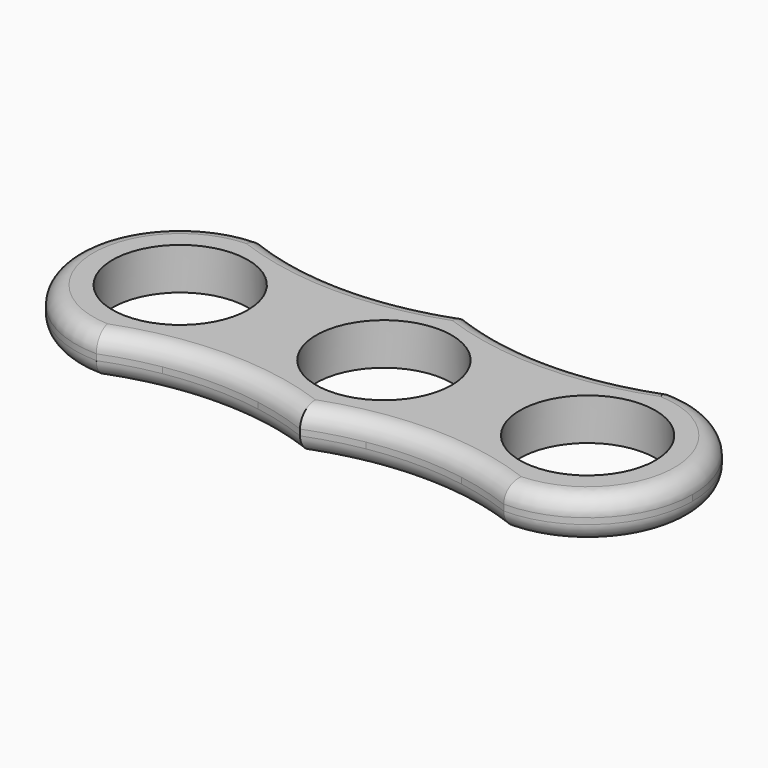
from build123d import *

# Parameters (mm, degrees)
F0_R         = 11.3
F1_DEPTH     = 7
F2_T2_ANGLE  = 60.8488693261
F2_T4_ANGLE  = 229.1896473945
F2_T6_ANGLE  = 60.8488693261
F2_T8_ANGLE  = 60.8488693262
F2_T10_ANGLE = 229.1896473945
F2_T12_ANGLE = 60.8488693262
F3_T2_ANGLE  = 60.8488693261
F3_T4_ANGLE  = 229.1896473945
F3_T6_ANGLE  = 60.8488693261
F3_T8_ANGLE  = 60.8488693262
F3_T10_ANGLE = 60.8488693262
F3_T12_ANGLE = 229.1896473945


# Not quite as in the source:
# - a fillet or chamfer that OpenCascade refuses, or shapes differently, is made with other operations: its cross-section is extruded or revolved along the edge and cut away or added


with BuildPart() as f1:
    # F0 (on Top) → F1 (new body)
    with BuildSketch(Plane.XY):
        with BuildLine():
            ThreePointArc((17, -4.1533119315), (17.3745503539, -2.0916500663), (17.5, 0))
            ThreePointArc((17.5, 0), (17.3745503539, 2.0916500663), (17, 4.1533119315))
            ThreePointArc((17, 4.1533119315), (16.5, 0), (17, -4.1533119315))
        make_face()
        with BuildLine():
            ThreePointArc((17, 4.1533119315), (17.3745503539, 2.0916500663), (17.5, 0))
            ThreePointArc((17.5, 0), (17.3745503539, -2.0916500663), (17, -4.1533119315))
            ThreePointArc((17, -4.1533119315), (19.903404144, -10.3699558954), (24.9737217118, -14.9925414878))
            ThreePointArc((24.9737217118, -14.9925414878), (29.5496426675, -16.0202705528), (34, -17.5))
            ThreePointArc((34, -17.5), (46.3743686708, -12.3743686708), (51.5, 0))
            ThreePointArc((51.5, 0), (46.3743686708, 12.3743686708), (34, 17.5))
            ThreePointArc((34, 17.5), (29.5496426675, 16.0202705528), (24.9737217118, 14.9925414878))
            ThreePointArc((24.9737217118, 14.9925414878), (19.903404144, 10.3699558954), (17, 4.1533119315))
        make_face()
        with Locations((34, 0)):
            Circle(F0_R, mode=Mode.SUBTRACT)
        with BuildLine():
            ThreePointArc((17, -4.1533119315), (16.5, 0), (17, 4.1533119315))
            ThreePointArc((17, 4.1533119315), (14.096595856, 10.3699558954), (9.0262782882, 14.9925414878))
            ThreePointArc((9.0262782882, 14.9925414878), (4.4503573325, 16.0202705528), (0, 17.5))
            ThreePointArc((0, 17.5), (-4.4503573325, 16.0202705528), (-9.0262782882, 14.9925414878))
            ThreePointArc((-9.0262782882, 14.9925414878), (-14.096595856, 10.3699558954), (-17, 4.1533119315))
            ThreePointArc((-17, 4.1533119315), (-16.6254496461, 2.0916500663), (-16.5, 0))
            ThreePointArc((-16.5, 0), (-16.6254496461, -2.0916500663), (-17, -4.1533119315))
            ThreePointArc((-17, -4.1533119315), (-14.096595856, -10.3699558954), (-9.0262782882, -14.9925414878))
            ThreePointArc((-9.0262782882, -14.9925414878), (-4.4503573325, -16.0202705528), (0, -17.5))
            ThreePointArc((0, -17.5), (4.4503573325, -16.0202705528), (9.0262782882, -14.9925414878))
            ThreePointArc((9.0262782882, -14.9925414878), (14.096595856, -10.3699558954), (17, -4.1533119315))
        make_face()
        Circle(F0_R, mode=Mode.SUBTRACT)
        with BuildLine():
            ThreePointArc((9.0262782882, 14.9925414878), (14.096595856, 10.3699558954), (17, 4.1533119315))
            ThreePointArc((17, 4.1533119315), (19.903404144, 10.3699558954), (24.9737217118, 14.9925414878))
            ThreePointArc((24.9737217118, 14.9925414878), (17, 14.3095450998), (9.0262782882, 14.9925414878))
        make_face()
        with BuildLine():
            ThreePointArc((24.9737217118, -14.9925414878), (19.903404144, -10.3699558954), (17, -4.1533119315))
            ThreePointArc((17, -4.1533119315), (14.096595856, -10.3699558954), (9.0262782882, -14.9925414878))
            ThreePointArc((9.0262782882, -14.9925414878), (17, -14.3095450998), (24.9737217118, -14.9925414878))
        make_face()
        with BuildLine():
            ThreePointArc((-17, 4.1533119315), (-14.096595856, 10.3699558954), (-9.0262782882, 14.9925414878))
            ThreePointArc((-9.0262782882, 14.9925414878), (-17, 14.3095450998), (-24.9737217118, 14.9925414878))
            ThreePointArc((-24.9737217118, 14.9925414878), (-19.903404144, 10.3699558954), (-17, 4.1533119315))
        make_face()
        with BuildLine():
            ThreePointArc((-24.9737217118, -14.9925414878), (-17, -14.3095450998), (-9.0262782882, -14.9925414878))
            ThreePointArc((-9.0262782882, -14.9925414878), (-14.096595856, -10.3699558954), (-17, -4.1533119315))
            ThreePointArc((-17, -4.1533119315), (-19.903404144, -10.3699558954), (-24.9737217118, -14.9925414878))
        make_face()
        with BuildLine():
            ThreePointArc((-16.5, 0), (-16.6254496461, 2.0916500663), (-17, 4.1533119315))
            ThreePointArc((-17, 4.1533119315), (-17.5, 0), (-17, -4.1533119315))
            ThreePointArc((-17, -4.1533119315), (-16.6254496461, -2.0916500663), (-16.5, 0))
        make_face()
        with BuildLine():
            ThreePointArc((-17, -4.1533119315), (-17.5, 0), (-17, 4.1533119315))
            ThreePointArc((-17, 4.1533119315), (-19.903404144, 10.3699558954), (-24.9737217118, 14.9925414878))
            ThreePointArc((-24.9737217118, 14.9925414878), (-29.5496426675, 16.0202705528), (-34, 17.5))
            ThreePointArc((-34, 17.5), (-51.5, 0), (-34, -17.5))
            ThreePointArc((-34, -17.5), (-29.5496426675, -16.0202705528), (-24.9737217118, -14.9925414878))
            ThreePointArc((-24.9737217118, -14.9925414878), (-19.903404144, -10.3699558954), (-17, -4.1533119315))
        make_face()
        with Locations((-34, 0)):
            Circle(F0_R, mode=Mode.SUBTRACT)
    extrude(amount=F1_DEPTH)

    # F2: fillet of radius 3 on 6 edges, made by hand

    # F2_s1 → F2_t2 (revolve, cut)
    with BuildSketch(Plane(origin=(-39.3629213467, -23.1166596288, 0), x_dir=(0, 0, 1), z_dir=(-0.8622977849, -0.5064015503, 0))):
        with BuildLine():
            ThreePointArc((4, 2.7261224717), (6.1213203436, 3.6048021282), (7, 5.7261224717))
            Line((7, 5.7261224717), (7, 2.7261224717))
            Line((7, 2.7261224717), (4, 2.7261224717))
        make_face()
    revolve(axis=Axis((-17, -61.1961195589, 7), (0, 0, -1)), revolution_arc=F2_T2_ANGLE, mode=Mode.SUBTRACT)

    # F2_s3 → F2_t4 (revolve, cut)
    with BuildSketch(Plane(origin=(-28.110475333, 12.8669086371, 0), x_dir=(0, 0, 1), z_dir=(0.9092737136, -0.416198647, 0))):
        with BuildLine():
            ThreePointArc((4, -3.3492460032), (6.1213203436, -2.4705663467), (7, -0.3492460032))
            Line((7, -0.3492460032), (7, -3.3492460032))
            Line((7, -3.3492460032), (4, -3.3492460032))
        make_face()
    revolve(axis=Axis((-34, 0, 7), (0, 0, 1)), revolution_arc=F2_T4_ANGLE, mode=Mode.SUBTRACT)

    # F2_s5 → F2_t6 (revolve, cut)
    with BuildSketch(Plane(origin=(14.0819673704, 8.2699158362, 0), x_dir=(0, 0, 1), z_dir=(0.8622977849, 0.5064015503, 0))):
        with BuildLine():
            ThreePointArc((4, -14.4915302372), (6.1213203436, -13.6128505808), (7, -11.4915302372))
            Line((7, -11.4915302372), (7, -14.4915302372))
            Line((7, -14.4915302372), (4, -14.4915302372))
        make_face()
    revolve(axis=Axis((-17, 61.1961195589, 7), (0, 0, -1)), revolution_arc=F2_T6_ANGLE, mode=Mode.SUBTRACT)

    # F2_s7 → F2_t8 (revolve, cut)
    with BuildSketch(Plane(origin=(39.3629213467, 23.1166596288, 0), x_dir=(0, 0, 1), z_dir=(0.8622977849, 0.5064015503, 0))):
        with BuildLine():
            ThreePointArc((4, 2.7261224717), (6.1213203436, 3.6048021282), (7, 5.7261224717))
            Line((7, 5.7261224717), (7, 2.7261224717))
            Line((7, 2.7261224717), (4, 2.7261224717))
        make_face()
    revolve(axis=Axis((17, 61.1961195588, 7), (0, 0, -1)), revolution_arc=F2_T8_ANGLE, mode=Mode.SUBTRACT)

    # F2_s9 → F2_t10 (revolve, cut)
    with BuildSketch(Plane(origin=(28.110475333, -12.8669086371, 0), x_dir=(0, 0, 1), z_dir=(-0.9092737136, 0.416198647, 0))):
        with BuildLine():
            ThreePointArc((4, -3.3492460032), (6.1213203436, -2.4705663467), (7, -0.3492460032))
            Line((7, -0.3492460032), (7, -3.3492460032))
            Line((7, -3.3492460032), (4, -3.3492460032))
        make_face()
    revolve(axis=Axis((34, 0, 7), (0, 0, 1)), revolution_arc=F2_T10_ANGLE, mode=Mode.SUBTRACT)

    # F2_s11 → F2_t12 (revolve, cut)
    with BuildSketch(Plane(origin=(-14.0819673704, -8.2699158362, 0), x_dir=(0, 0, 1), z_dir=(-0.8622977849, -0.5064015503, 0))):
        with BuildLine():
            ThreePointArc((4, -14.4915302372), (6.1213203436, -13.6128505808), (7, -11.4915302372))
            Line((7, -11.4915302372), (7, -14.4915302372))
            Line((7, -14.4915302372), (4, -14.4915302372))
        make_face()
    revolve(axis=Axis((17, -61.1961195588, 7), (0, 0, -1)), revolution_arc=F2_T12_ANGLE, mode=Mode.SUBTRACT)

    # F3: fillet of radius 3 on 6 edges, made by hand

    # F3_s1 → F3_t2 (revolve, cut)
    with BuildSketch(Plane(origin=(-39.3629213467, -23.1166596288, 0), x_dir=(0, 0, 1), z_dir=(-0.8622977849, -0.5064015503, 0))):
        with BuildLine():
            ThreePointArc((0, 5.7261224717), (0.8786796564, 3.6048021282), (3, 2.7261224717))
            Line((3, 2.7261224717), (0, 2.7261224717))
            Line((0, 2.7261224717), (0, 5.7261224717))
        make_face()
    revolve(axis=Axis((-17, -61.1961195589, 0), (0, 0, -1)), revolution_arc=F3_T2_ANGLE, mode=Mode.SUBTRACT)

    # F3_s3 → F3_t4 (revolve, cut)
    with BuildSketch(Plane(origin=(-28.110475333, 12.8669086371, 0), x_dir=(0, 0, 1), z_dir=(0.9092737136, -0.416198647, 0))):
        with BuildLine():
            ThreePointArc((0, -0.3492460032), (0.8786796564, -2.4705663467), (3, -3.3492460032))
            Line((3, -3.3492460032), (0, -3.3492460032))
            Line((0, -3.3492460032), (0, -0.3492460032))
        make_face()
    revolve(axis=Axis((-34, 0, 0), (0, 0, 1)), revolution_arc=F3_T4_ANGLE, mode=Mode.SUBTRACT)

    # F3_s5 → F3_t6 (revolve, cut)
    with BuildSketch(Plane(origin=(14.0819673704, 8.2699158362, 0), x_dir=(0, 0, 1), z_dir=(0.8622977849, 0.5064015503, 0))):
        with BuildLine():
            ThreePointArc((0, -11.4915302372), (0.8786796564, -13.6128505808), (3, -14.4915302372))
            Line((3, -14.4915302372), (0, -14.4915302372))
            Line((0, -14.4915302372), (0, -11.4915302372))
        make_face()
    revolve(axis=Axis((-17, 61.1961195589, 0), (0, 0, -1)), revolution_arc=F3_T6_ANGLE, mode=Mode.SUBTRACT)

    # F3_s7 → F3_t8 (revolve, cut)
    with BuildSketch(Plane(origin=(39.3629213467, 23.1166596288, 0), x_dir=(0, 0, 1), z_dir=(0.8622977849, 0.5064015503, 0))):
        with BuildLine():
            ThreePointArc((0, 5.7261224717), (0.8786796564, 3.6048021282), (3, 2.7261224717))
            Line((3, 2.7261224717), (0, 2.7261224717))
            Line((0, 2.7261224717), (0, 5.7261224717))
        make_face()
    revolve(axis=Axis((17, 61.1961195588, 0), (0, 0, -1)), revolution_arc=F3_T8_ANGLE, mode=Mode.SUBTRACT)

    # F3_s9 → F3_t10 (revolve, cut)
    with BuildSketch(Plane(origin=(-14.0819673704, -8.2699158362, 0), x_dir=(0, 0, 1), z_dir=(-0.8622977849, -0.5064015503, 0))):
        with BuildLine():
            ThreePointArc((0, -11.4915302372), (0.8786796564, -13.6128505808), (3, -14.4915302372))
            Line((3, -14.4915302372), (0, -14.4915302372))
            Line((0, -14.4915302372), (0, -11.4915302372))
        make_face()
    revolve(axis=Axis((17, -61.1961195588, 0), (0, 0, -1)), revolution_arc=F3_T10_ANGLE, mode=Mode.SUBTRACT)

    # F3_s11 → F3_t12 (revolve, cut)
    with BuildSketch(Plane(origin=(28.110475333, -12.8669086371, 0), x_dir=(0, 0, 1), z_dir=(-0.9092737136, 0.416198647, 0))):
        with BuildLine():
            ThreePointArc((3, -3.3492460032), (0.8786796564, -2.4705663467), (0, -0.3492460032))
            Line((0, -0.3492460032), (0, -3.3492460032))
            Line((0, -3.3492460032), (3, -3.3492460032))
        make_face()
    revolve(axis=Axis((34, 0, 0), (0, 0, 1)), revolution_arc=F3_T12_ANGLE, mode=Mode.SUBTRACT)


solid = f1.part
